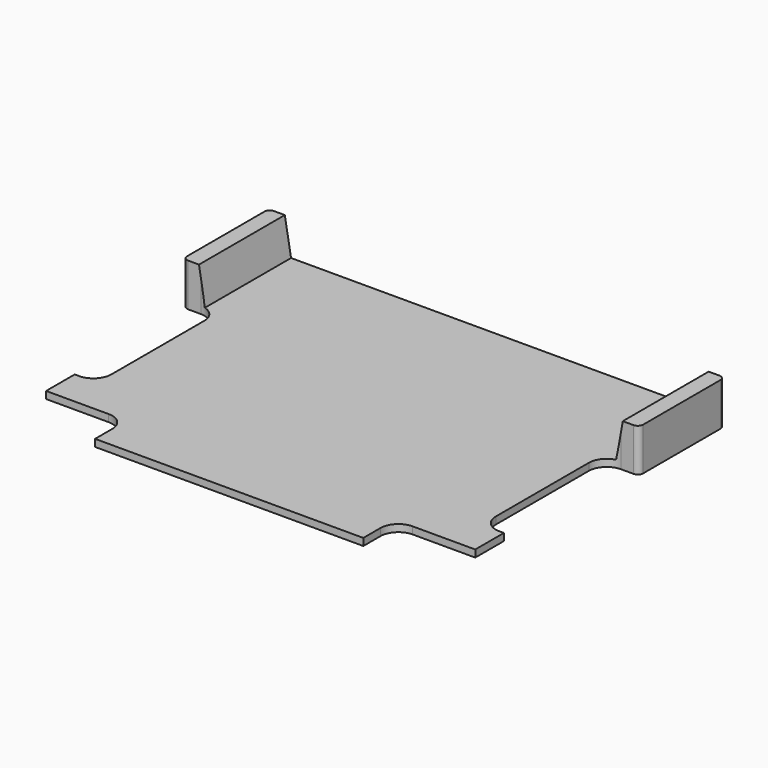
from build123d import *

# Parameters (mm, degrees)
F0_W     = 15
F0_H     = 1
F0_H_2   = 1.2
F0_W_2   = 1.1
F0_H_3   = 6
F0_W_3   = 0.9
F5_DEPTH = 6
F6_R     = 1
F7_R     = 0.3


with BuildPart() as f2:
    # F2: sweep along a path in F1
    with BuildLine(Plane.XZ) as f2_path:
        Line((0, 0), (0, 0.4))
    # F0 (on Top) → F2 (sweep)
    with BuildSketch(Plane.XY):
        Polygon((-10.75, 1), (-10.75, 0), (-7.5, 0), (7.5, 0), (10.75, 0), (10.75, 1), align=None)
        Polygon((-12, 0), (-10.75, 0), (-10.75, 1), (-10.75, 2), (-12, 2), align=None)
        with Locations((0, -0.5)):
            Rectangle(F0_W, F0_H)
        Polygon((-10.75, 2), (-10.75, 1), (10.75, 1), (10.75, 2), (10.75, 10.5), (10.75, 16.5), (-10.75, 16.5), (-10.75, 10.5), align=None)
        with Locations((0, -1.6)):
            Rectangle(F0_W, F0_H_2)
        Polygon((10.75, 2), (10.75, 1), (10.75, 0), (12, 0), (12, 2), align=None)
        with Locations((-11.3, 13.5)):
            Rectangle(F0_W_2, F0_H_3)
        with Locations((-12.3, 13.5)):
            Rectangle(F0_W_3, F0_H_3)
        with Locations((11.3, 13.5)):
            Rectangle(F0_W_2, F0_H_3)
        with Locations((12.3, 13.5)):
            Rectangle(F0_W_3, F0_H_3)
    sweep(path=f2_path.line)

    # F3: sweep along a path in F1
    with BuildLine(Plane.XZ) as f3_path:
        Line((0, 0), (0, 0.4))
        Line((0, 0.4), (0, 2.4))
    # F0 (on Top) → F3 (sweep)
    with BuildSketch(Plane.XY):
        with Locations((12.3, 13.5)):
            Rectangle(F0_W_3, F0_H_3)
        with Locations((-12.3, 13.5)):
            Rectangle(F0_W_3, F0_H_3)
    sweep(path=f3_path.line)

    # F4 (on face) → F5 (join, through all)
    with BuildSketch(Plane(origin=(0, 16.5, 0), x_dir=(-1, 0, 0), z_dir=(0, 1, 0))):
        Polygon((-11.5, 0.4), (-11.85, 2.4), (-11.85, 0.4), align=None)
        Polygon((11.85, 2.4), (11.5, 0.4), (11.85, 0.4), align=None)
    extrude(amount=-F5_DEPTH)

    # F6
    f6_edges = [f2.edges().sort_by_distance(p)[0] for p in [
        (7.5, 0, 0.2),
        (-7.5, 0, 0.2),
        (-10.75, 2, 0.2),
        (-10.75, 10.5, 0.2),
        (10.75, 10.5, 0.2),
        (10.75, 2, 0.2),
    ]]
    fillet(f6_edges, radius=F6_R)

    # F7
    f7_edges = [f2.edges().sort_by_distance(p)[0] for p in [
        (-12.75, 16.5, 1.2),
        (12.75, 16.5, 1.2),
        (12.75, 10.5, 1.2),
        (-12.75, 10.5, 1.2),
    ]]
    fillet(f7_edges, radius=F7_R)


solid = f2.part
